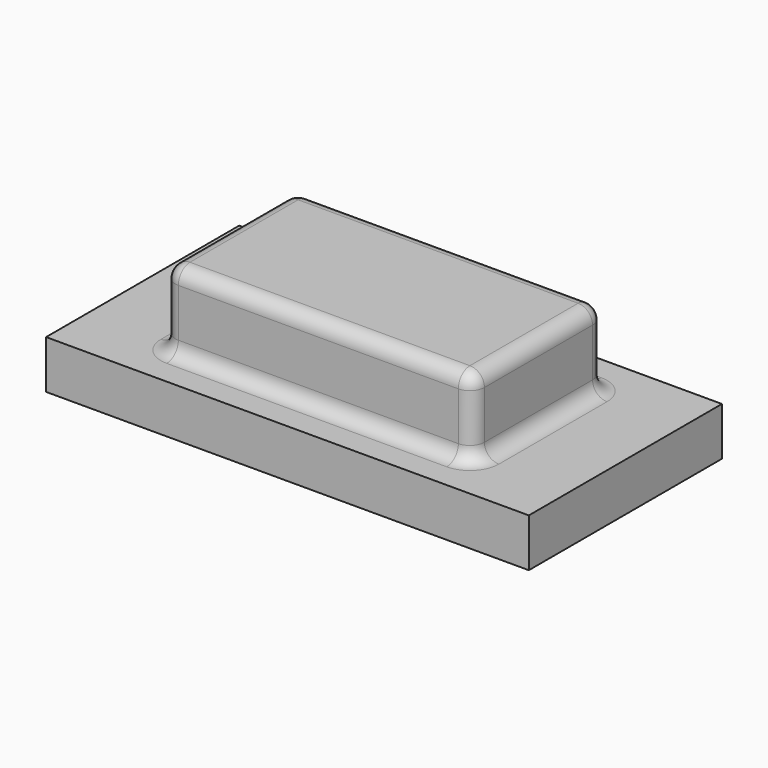
from build123d import *

# Parameters (mm, degrees)
F0_W     = 500
F0_H     = 250
F1_DEPTH = 25
F2_W     = 320
F2_H     = 170
F3_DEPTH = 80
F4_R     = 15


with BuildPart() as f1:
    # F0 (on Top) → F1 (new body, symmetric)
    with BuildSketch(Plane.XY):
        Rectangle(F0_W, F0_H)
    extrude(amount=F1_DEPTH, both=True)

    # F2 (on face) → F3 (join)
    with BuildSketch(Plane.XY.offset(25)):
        Rectangle(F2_W, F2_H)
    extrude(amount=F3_DEPTH)

    # F4
    f4_edges = [f1.edges().sort_by_distance(p)[0] for p in [
        (0, -85, 105),
        (-160, 0, 105),
        (160, 0, 105),
        (-160, -85, 65),
        (-160, 85, 65),
        (160, -85, 65),
        (0, 85, 105),
        (160, 85, 65),
        (0, -85, 25),
        (-160, 0, 25),
        (160, 0, 25),
        (0, 85, 25),
    ]]
    fillet(f4_edges, radius=F4_R)


solid = f1.part
